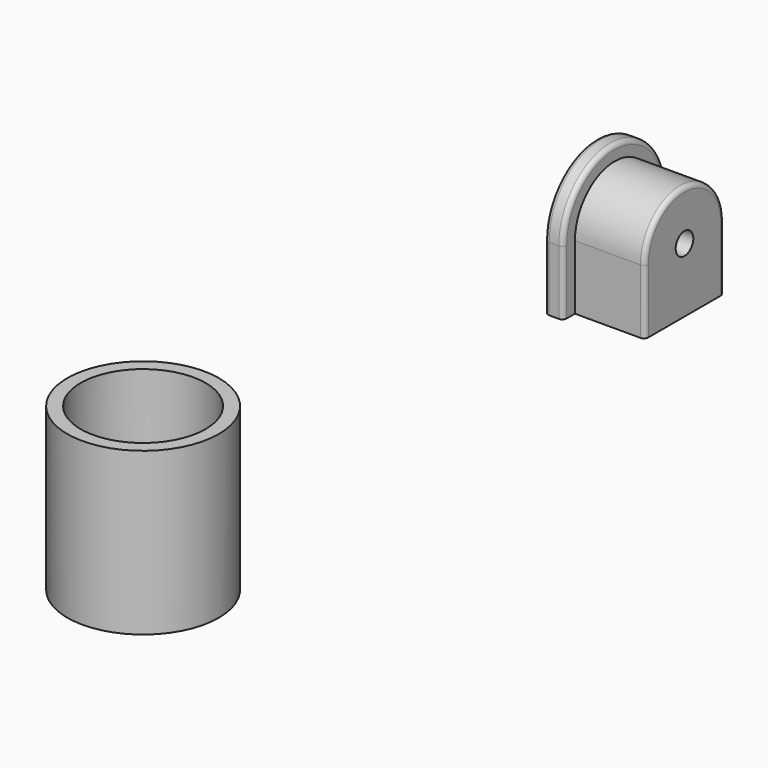
from build123d import *

# Parameters (mm, degrees)
F0_R     = 8.5
F1_DEPTH = 2
F0_R_2   = 10.3
F2_DEPTH = 22
F0_W     = 9.5
F0_H     = 5.25
F0_W_2   = 2.5
F0_H_2   = 1.5
F3_DEPTH = 8.75
F5_R     = 1.5
F6_DEPTH = 27.1577554153
F7_R     = 0.6
F8_D     = 6
F8_DEPTH = 5
F8_TIP   = 1.8025818571


with BuildPart() as f1:
    # F0 (on Top) → F1 (new body)
    with BuildSketch(Plane.XY):
        Circle(F0_R)
    extrude(amount=F1_DEPTH)

    # F0 (on Top) → F2 (join)
    with BuildSketch(Plane.XY):
        Circle(F0_R_2)
        Circle(F0_R, mode=Mode.SUBTRACT)
    extrude(amount=F2_DEPTH)


with BuildPart() as f3:
    # F0 (on Top) → F3 (new body)
    with BuildSketch(Plane.XY):
        with Locations((-9.6067554153, 102.2247694518)):
            Rectangle(F0_W, F0_H)
        Polygon((-16.8567554153, 99.5997694518), (-14.3567554153, 99.5997694518), (-14.3567554153, 104.8497694518), (-14.3567554153, 106.8497694518), (-16.8567554153, 106.8497694518), align=None)
        with Locations((-15.6067554153, 97.3497694518)):
            Rectangle(F0_W_2, F0_H_2)
        with Locations((-15.6067554153, 98.8497694518)):
            Rectangle(F0_W_2, F0_H_2)
        with Locations((-9.6067554153, 97.3497694518)):
            Rectangle(F0_W, F0_H_2)
        with Locations((-9.6067554153, 98.8497694518)):
            Rectangle(F0_W, F0_H_2)
        with Locations((-9.6067554153, 93.9747694518)):
            Rectangle(F0_W, F0_H)
        Polygon((-14.3567554153, 89.3497694518), (-14.3567554153, 91.3497694518), (-14.3567554153, 96.5997694518), (-16.8567554153, 96.5997694518), (-16.8567554153, 89.3497694518), align=None)
    extrude(amount=-F3_DEPTH)

    # F0 (on Top) → F4 (revolve)
    with BuildSketch(Plane.XY):
        with Locations((-9.6067554153, 97.3497694518)):
            Rectangle(F0_W, F0_H_2)
        with Locations((-15.6067554153, 97.3497694518)):
            Rectangle(F0_W_2, F0_H_2)
        Polygon((-14.3567554153, 89.3497694518), (-14.3567554153, 91.3497694518), (-14.3567554153, 96.5997694518), (-16.8567554153, 96.5997694518), (-16.8567554153, 89.3497694518), align=None)
        with Locations((-9.6067554153, 93.9747694518)):
            Rectangle(F0_W, F0_H)
    revolve(axis=Axis((-10.8567554153, 98.0997694518, 0), (1, 0, 0)))

    # F5 (on face) → F6 (cut, through all)
    with BuildSketch(Plane(origin=(-16.8567554153, 0, 0), x_dir=(0, -1, 0), z_dir=(-1, 0, 0))):
        with Locations((-98.0997694518, 0)):
            Circle(F5_R)
    extrude(amount=-F6_DEPTH, mode=Mode.SUBTRACT)

    # F7
    f7_edges = [f3.edges().sort_by_distance(p)[0] for p in [
        (-16.856755, 89.349769, -4.375),
        (-16.856755, 106.849769, -4.375),
        (-15.606755, 98.099769, -8.75),
        (-14.356755, 89.349769, -4.375),
        (-14.356755, 106.849769, -4.375),
        (-4.856755, 91.349769, -4.375),
        (-4.856755, 98.099769, 6.75),
        (-4.856755, 104.849769, -4.375),
        (-14.356755, 98.099769, 8.75),
        (-16.856755, 98.099769, 8.75),
    ]]
    fillet(f7_edges, radius=F7_R)

    # F8
    with Locations(Plane(origin=(-16.8567554153, 0, 0), x_dir=(0, -1, 0), z_dir=(-1, 0, 0))):
        with Locations((-98.0997694518, 0)):
            Hole(F8_D / 2, depth=F8_DEPTH)
            with Locations((0, 0, -(F8_DEPTH + F8_TIP / 2))):  # 118° drill point
                Cone(0, F8_D / 2, F8_TIP, mode=Mode.SUBTRACT)


solid = Compound([f1.part, f3.part])
